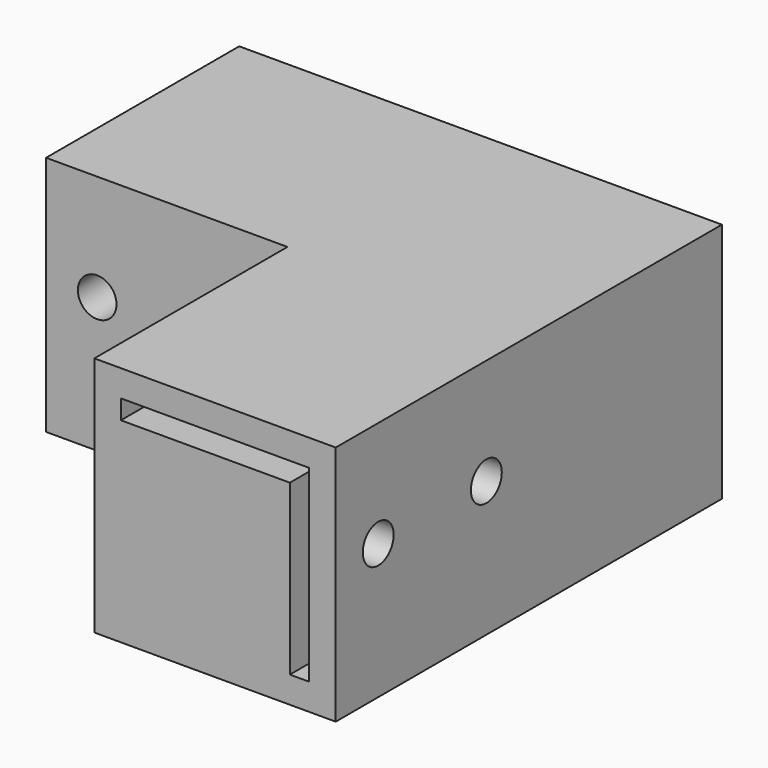
from build123d import *

# Parameters (mm, degrees)
F0_W      = 25
F0_H      = 25
F1_DEPTH  = 25
F2_DEPTH  = 25
F3_DEPTH  = 25
F4_W      = 25
F4_H      = 25
F5_DEPTH  = 25
F6_W      = 17.5
F6_H      = 2
F6_W_2    = 2
F6_H_2    = 17.5
F7_DEPTH  = 25
F8_W      = 2
F8_H      = 2
F8_W_2    = 17.5
F8_H_2    = 17.5
F9_DEPTH  = 25
F10_R     = 2
F11_DEPTH = 25
F12_R     = 2
F13_DEPTH = 25


# Not quite as in the source:
# - a feature names something its author has since deleted; it is built from what else it names


with BuildPart() as f1:
    # F0 (on Top) → F1 (new body)
    with BuildSketch(Plane.XY):
        with Locations((12.5, 12.5)):
            Rectangle(F0_W, F0_H)
    extrude(amount=F1_DEPTH)

    # F2 (add): a face of the model
    f2_faces = [f1.faces().sort_by_distance(p)[0] for p in [
        (12.5, 0, 12.5),
    ]]
    extrude(f2_faces, amount=F2_DEPTH)

    # F3 (add): a face of the model
    f3_faces = [f1.faces().sort_by_distance(p)[0] for p in [
        (0, 0, 12.5),
    ]]
    extrude(f3_faces, amount=F3_DEPTH)

    # F4 (on face) → F5 (cut)
    with BuildSketch(Plane.XY.offset(25)):
        with Locations((-12.5, -12.5)):
            Rectangle(F4_W, F4_H)
    extrude(amount=-F5_DEPTH, mode=Mode.SUBTRACT)

    # F6 (on face) → F7 (cut)
    with BuildSketch(Plane.XZ.offset(25)):
        with Locations((11.5, 21.25)):
            Rectangle(F6_W, F6_H)
        with Locations((21.25, 21.25)):
            Rectangle(F6_W_2, F6_H)
        with Locations((21.25, 11.5)):
            Rectangle(F6_W_2, F6_H_2)
    extrude(amount=-F7_DEPTH, mode=Mode.SUBTRACT)

    # F8 (on face) → F9 (cut)
    with BuildSketch(Plane(origin=(-25, 0, 0), x_dir=(0, -1, 0), z_dir=(-1, 0, 0))):
        with Locations((-21.25, 21.25)):
            Rectangle(F8_W, F8_H)
        with Locations((-11.5, 21.25)):
            Rectangle(F8_W_2, F8_H)
        with Locations((-21.25, 11.5)):
            Rectangle(F8_W, F8_H_2)
    extrude(amount=-F9_DEPTH, mode=Mode.SUBTRACT)

    # F10 (on face) → F11 (cut)
    with BuildSketch(Plane(origin=(0, 25, 0), x_dir=(-1, 0, 0), z_dir=(0, 1, 0))):
        with Locations((19.7084973779, 14)):
            Circle(F10_R)
        with Locations((5.5, 14)):
            Circle(F10_R)
    extrude(amount=-F11_DEPTH, mode=Mode.SUBTRACT)

    # F12 (on face) → F13 (cut)
    with BuildSketch(Plane.YZ.offset(25)):
        with Locations((-19.5, 14)):
            Circle(F12_R)
        with Locations((-5.5, 14)):
            Circle(F12_R)
    extrude(amount=-F13_DEPTH, mode=Mode.SUBTRACT)


solid = f1.part
